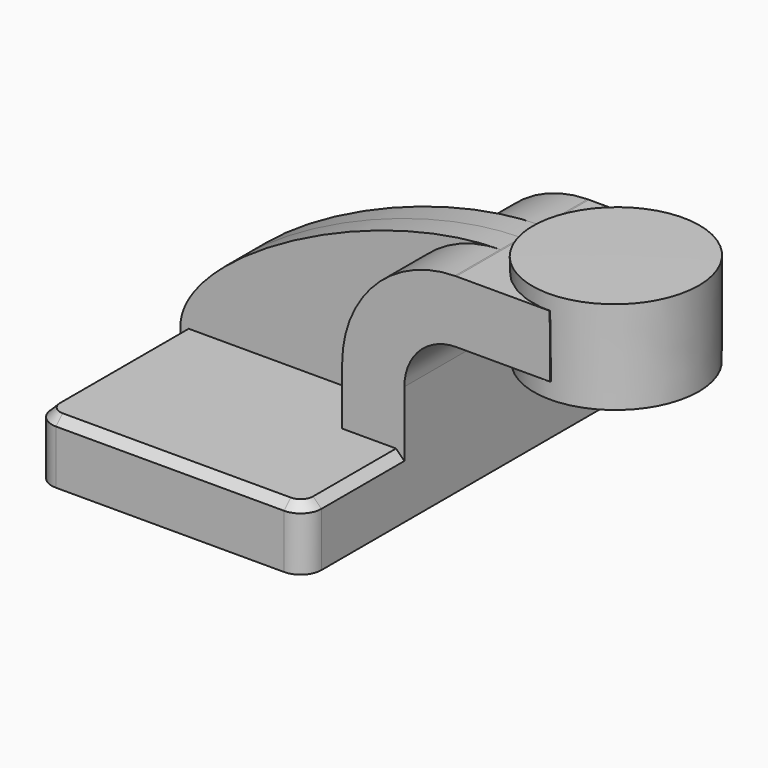
from build123d import *

# Parameters (mm, degrees)
F1_DEPTH     = 63.5
F2_DEPTH     = 25.4
F3_DEPTH     = 7.9375
F5_R         = 6.35
F7_T1_DEPTH  = 69.85
F7_T3_DEPTH  = 31.75
F7_T5_DEPTH  = 49.2125
F7_T7_DEPTH  = 31.75
F7_T9_DEPTH  = 49.2125
F7_T12_ANGLE = 90
F7_T14_ANGLE = 90
F7_T16_ANGLE = 90
F7_T18_ANGLE = 90


# Not quite as in the source:
# - a fillet or chamfer that OpenCascade refuses, or shapes differently, is made with other operations: its cross-section is extruded or revolved along the edge and cut away or added
# - a feature of the source that left no trace in its solid (it failed there, or was rolled back) is left out


with BuildPart() as f1:
    # F0 (on Front) → F1 (new body, symmetric)
    with BuildSketch(Plane.XZ):
        Polygon((22.225, 9.525), (-41.275, 9.525), (-41.275, -9.525), (41.275, -9.525), (41.275, 9.525), align=None)
    extrude(amount=F1_DEPTH, both=True)

    # F0 (on Front) → F2 (join, symmetric)
    with BuildSketch(Plane.XZ):
        with BuildLine():
            Line((22.225, 27.0002), (22.225, 9.525))
            Line((22.225, 9.525), (41.275, 9.525))
            Line((41.275, 9.525), (41.275, 27.0002))
            ThreePointArc((41.275, 27.0002), (45.9246798487, 38.2255201513), (57.15, 42.8752))
            Line((57.15, 42.8752), (60.325, 42.8752))
            Line((60.325, 42.8752), (60.325, 61.9252))
            Line((60.325, 61.9252), (57.15, 61.9252))
            add(Edge.make_bspline(
                [(56.7267505246, 61.9226352656), (56.8680376244, 61.9238665385), (57.0091218232, 61.9247220333), (57.15, 61.9252)],
                knots=[111.1164220424, 111.1164220424, 111.1164220424, 111.1164220424, 111.5045361635, 111.5045361635, 111.5045361635, 111.5045361635], degree=3))
            ThreePointArc((56.7267505246, 61.9226352656), (32.3051050221, 51.5458069091), (22.225, 27.0002))
        make_face()
        Polygon((85.769072175, 61.9252), (60.325, 61.9252), (60.325, 42.8752), (85.9264696617, 42.8752), align=None)
    extrude(amount=F2_DEPTH, both=True)

    # F0 (on Front) → F3 (join, symmetric)
    with BuildSketch(Plane.XZ):
        with BuildLine():
            add(Edge.make_bspline(
                [(-41.275, 9.525), (-40.8048993717, 30.4163066823), (16.2764907719, 61.5701239012), (56.7267505246, 61.9226352656)],
                knots=[0, 0, 0, 0, 111.1164220424, 111.1164220424, 111.1164220424, 111.1164220424], degree=3))
            Line((-41.275, 9.525), (22.225, 9.525))
            Line((22.225, 9.525), (22.225, 27.0002))
            ThreePointArc((22.225, 27.0002), (32.3051050221, 51.5458069091), (56.7267505246, 61.9226352656))
        make_face()
    extrude(amount=F3_DEPTH, both=True)

    # F5
    f5_edges = [f1.edges().sort_by_distance(p)[0] for p in [
        (-41.275, 63.5, 0),
        (-41.275, -63.5, 0),
        (41.275, -63.5, 0),
        (41.275, 63.5, 0),
    ]]
    fillet(f5_edges, radius=F5_R)

    # F7: chamfer of 2.54 on 10 edges, made by hand

    # F7_s2 → F7_t1 (cut)
    with BuildSketch(Plane.YZ.offset(-34.925)):
        Polygon((60.96, 9.525), (63.5, 6.985), (63.5, 9.525), align=None)
        Polygon((-60.96, 9.525), (-63.5, 6.985), (-63.5, 9.525), align=None)
    extrude(amount=F7_T1_DEPTH, mode=Mode.SUBTRACT)

    # F7_s4 → F7_t3 (cut)
    with BuildSketch(Plane.XZ.offset(-57.15)):
        Polygon((38.735, 9.525), (41.275, 6.985), (41.275, 9.525), align=None)
    extrude(amount=F7_T3_DEPTH, mode=Mode.SUBTRACT)

    # F7_s6 → F7_t5 (cut)
    with BuildSketch(Plane.XZ.offset(-57.15)):
        Polygon((-38.735, 9.525), (-41.275, 6.985), (-41.275, 9.525), align=None)
    extrude(amount=F7_T5_DEPTH, mode=Mode.SUBTRACT)

    # F7_s8 → F7_t7 (cut)
    with BuildSketch(Plane.XZ.offset(25.4)):
        Polygon((41.275, 6.985), (38.735, 9.525), (41.275, 9.525), align=None)
    extrude(amount=F7_T7_DEPTH, mode=Mode.SUBTRACT)

    # F7_s10 → F7_t9 (cut)
    with BuildSketch(Plane.XZ.offset(7.9375)):
        Polygon((-41.275, 6.985), (-38.735, 9.525), (-41.275, 9.525), align=None)
    extrude(amount=F7_T9_DEPTH, mode=Mode.SUBTRACT)

    # F7_s11 → F7_t12 (revolve, cut)
    with BuildSketch(Plane.XZ.offset(-57.15)):
        Polygon((38.735, 9.525), (41.275, 6.985), (41.275, 9.525), align=None)
    revolve(axis=Axis((34.925, 57.15, 9.525), (0, 0, 1)), revolution_arc=F7_T12_ANGLE, mode=Mode.SUBTRACT)

    # F7_s13 → F7_t14 (revolve, cut)
    with BuildSketch(Plane.XZ.offset(-57.15)):
        Polygon((-38.735, 9.525), (-41.275, 6.985), (-41.275, 9.525), align=None)
    revolve(axis=Axis((-34.925, 57.15, 9.525), (0, 0, -1)), revolution_arc=F7_T14_ANGLE, mode=Mode.SUBTRACT)

    # F7_s15 → F7_t16 (revolve, cut)
    with BuildSketch(Plane.XZ.offset(57.15)):
        Polygon((41.275, 6.985), (38.735, 9.525), (41.275, 9.525), align=None)
    revolve(axis=Axis((34.925, -57.15, 9.525), (0, 0, -1)), revolution_arc=F7_T16_ANGLE, mode=Mode.SUBTRACT)

    # F7_s17 → F7_t18 (revolve, cut)
    with BuildSketch(Plane.XZ.offset(57.15)):
        Polygon((-38.735, 9.525), (-41.275, 6.985), (-41.275, 9.525), align=None)
    revolve(axis=Axis((-34.925, -57.15, 9.525), (0, 0, 1)), revolution_arc=F7_T18_ANGLE, mode=Mode.SUBTRACT)


with BuildPart() as f4:
    # F0 (on Front) → F4 (revolve)
    with BuildSketch(Plane.XZ):
        Polygon((85.769072175, 66.675), (85.769072175, 61.9252), (85.9264696617, 42.8752), (85.965923965, 38.1), (111.125, 38.1), (111.125, 66.675), align=None)
    revolve(axis=Axis((85.86749807, 0, 50.0126), (0.0082620533, 0, -0.9999658687)))


solid = Compound([f1.part, f4.part])
